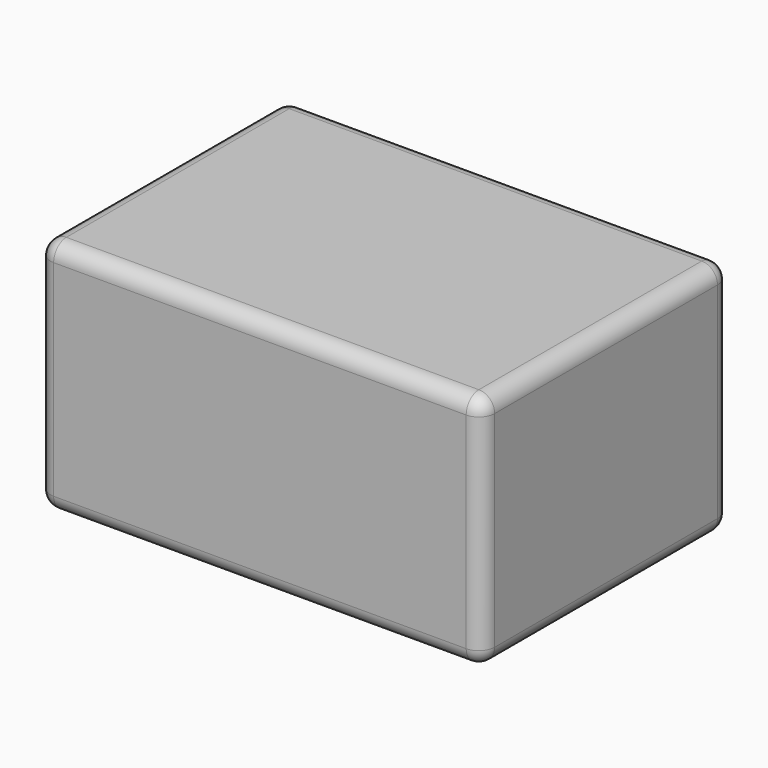
from build123d import *

# Parameters (mm, degrees)
F0_W         = 140.3584312648
F0_H         = 98.0234518647
F1_DEPTH     = 25
F2_DEPTH     = 50
F3_DEPTH     = 25
F4_R         = 5
F5_T1_DEPTH  = 65
F5_S5_W      = 5
F5_S5_H      = 5
F5_T6_DEPTH  = 5
F5_S11_W     = 5
F5_S11_H     = 5
F5_T12_DEPTH = 5
F5_S17_W     = 5
F5_S17_H     = 5
F5_T18_DEPTH = 5
F5_S23_W     = 5
F5_S23_H     = 5
F5_T24_DEPTH = 5
F5_S29_W     = 5
F5_S29_H     = 5
F5_T30_DEPTH = 5
F5_S35_W     = 5
F5_S35_H     = 5
F5_T36_DEPTH = 5
F5_S41_W     = 5
F5_S41_H     = 5
F5_T42_DEPTH = 5
F5_S47_W     = 5
F5_S47_H     = 5
F5_T48_DEPTH = 5


# Not quite as in the source:
# - a fillet or chamfer that OpenCascade refuses, or shapes differently, is made with other operations: its cross-section is extruded or revolved along the edge and cut away or added


with BuildPart() as f1:
    # F0 (on Top) → F1 (new body)
    with BuildSketch(Plane.XY):
        with Locations((-51.4516541734, -13.0883678794)):
            Rectangle(F0_W, F0_H)
    extrude(amount=F1_DEPTH)

    # F2 (add): a face of the model
    f2_faces = [f1.faces().sort_by_distance(p)[0] for p in [
        (-51.4516541734, -13.0883678794, 0),
    ]]
    extrude(f2_faces, amount=F2_DEPTH)

    # F3 (add): a face of the model
    f3_faces = [f1.faces().sort_by_distance(p)[0] for p in [
        (-51.4516541734, -13.0883678794, -50),
    ]]
    extrude(f3_faces, amount=-F3_DEPTH)

    # F4
    f4_edges = [f1.edges().sort_by_distance(p)[0] for p in [
        (18.727561, -13.088368, 25),
        (-121.63087, -13.088368, 25),
        (-51.451654, 35.923358, 25),
        (-51.451654, -62.100094, 25),
        (-51.451654, 35.923358, -50),
        (-121.63087, -13.088368, -50),
        (-51.451654, -62.100094, -50),
        (18.727561, -13.088368, -50),
    ]]
    fillet(f4_edges, radius=F4_R)

    # F5: fillet of radius 5 on 4 edges, made by hand

    # F5_s2 → F5_t1 (cut)
    with BuildSketch(Plane.XY.offset(-45)):
        with BuildLine():
            ThreePointArc((-116.6308698058, 35.923358053), (-120.1664037117, 34.4588919589), (-121.6308698058, 30.923358053))
            Line((-121.6308698058, 30.923358053), (-121.6308698058, 35.923358053))
            Line((-121.6308698058, 35.923358053), (-116.6308698058, 35.923358053))
        make_face()
        with BuildLine():
            ThreePointArc((13.7275614589, 35.923358053), (17.2630953649, 34.4588919589), (18.7275614589, 30.923358053))
            Line((18.7275614589, 30.923358053), (18.7275614589, 35.923358053))
            Line((18.7275614589, 35.923358053), (13.7275614589, 35.923358053))
        make_face()
        with BuildLine():
            ThreePointArc((18.7275614589, -57.1000938118), (17.2630953649, -60.6356277177), (13.7275614589, -62.1000938118))
            Line((13.7275614589, -62.1000938118), (18.7275614589, -62.1000938118))
            Line((18.7275614589, -62.1000938118), (18.7275614589, -57.1000938118))
        make_face()
        with BuildLine():
            ThreePointArc((-121.6308698058, -57.1000938118), (-120.1664037117, -60.6356277177), (-116.6308698058, -62.1000938118))
            Line((-116.6308698058, -62.1000938118), (-121.6308698058, -62.1000938118))
            Line((-121.6308698058, -62.1000938118), (-121.6308698058, -57.1000938118))
        make_face()
    extrude(amount=F5_T1_DEPTH, mode=Mode.SUBTRACT)


with BuildPart() as f5_tool4:
    # F5_s5 → F5_t6 (new body)
    with BuildSketch(Plane.YZ.offset(-116.6308698058)):
        with Locations((-59.6000938118, -47.5)):
            Rectangle(F5_S5_W, F5_S5_H)
    extrude(amount=-F5_T6_DEPTH)

    # F5_s7 → F5_t8 (revolve, cut)
    with BuildSketch(Plane(origin=(-116.6308698058, -57.1000938118, -45), x_dir=(0, 0.7071067812, 0.7071067812), z_dir=(0, -0.7071067812, 0.7071067812))):
        with BuildLine():
            ThreePointArc((0, -5), (5, 0), (0, 5))
            Line((0, 5), (0, -5))
        make_face()
    revolve(axis=Axis((-116.6308698058, -57.1000938118, -45), (-1, 0, 0)), mode=Mode.SUBTRACT)


with BuildPart() as f1_1:
    add(f1.part)

    # F5_t3: cut F5_tool4
    add(f5_tool4.part, mode=Mode.SUBTRACT)


with BuildPart() as f5_tool10:
    # F5_s11 → F5_t12 (new body)
    with BuildSketch(Plane.YZ.offset(-116.6308698058)):
        with Locations((-59.6000938118, 22.5)):
            Rectangle(F5_S11_W, F5_S11_H)
    extrude(amount=-F5_T12_DEPTH)

    # F5_s13 → F5_t14 (revolve, cut)
    with BuildSketch(Plane(origin=(-116.6308698058, -57.1000938118, 20), x_dir=(0, 0.7071067812, -0.7071067812), z_dir=(0, 0.7071067812, 0.7071067812))):
        with BuildLine():
            ThreePointArc((0, -5), (5, 0), (0, 5))
            Line((0, 5), (0, -5))
        make_face()
    revolve(axis=Axis((-116.6308698058, -57.1000938118, 20), (-1, 0, 0)), mode=Mode.SUBTRACT)


with BuildPart() as f1_2:
    add(f1_1.part)

    # F5_t9: cut F5_tool10
    add(f5_tool10.part, mode=Mode.SUBTRACT)


with BuildPart() as f5_tool16:
    # F5_s17 → F5_t18 (new body)
    with BuildSketch(Plane.YZ.offset(13.7275614589)):
        with Locations((-59.6000938118, 22.5)):
            Rectangle(F5_S17_W, F5_S17_H)
    extrude(amount=F5_T18_DEPTH)

    # F5_s19 → F5_t20 (revolve, cut)
    with BuildSketch(Plane(origin=(13.7275614589, -57.1000938118, 20), x_dir=(0, 0.7071067812, -0.7071067812), z_dir=(0, -0.7071067812, -0.7071067812))):
        with BuildLine():
            ThreePointArc((0, -5), (5, 0), (0, 5))
            Line((0, 5), (0, -5))
        make_face()
    revolve(axis=Axis((13.7275614589, -57.1000938118, 20), (1, 0, 0)), mode=Mode.SUBTRACT)


with BuildPart() as f1_3:
    add(f1_2.part)

    # F5_t15: cut F5_tool16
    add(f5_tool16.part, mode=Mode.SUBTRACT)


with BuildPart() as f5_tool22:
    # F5_s23 → F5_t24 (new body)
    with BuildSketch(Plane.YZ.offset(13.7275614589)):
        with Locations((-59.6000938118, -47.5)):
            Rectangle(F5_S23_W, F5_S23_H)
    extrude(amount=F5_T24_DEPTH)

    # F5_s25 → F5_t26 (revolve, cut)
    with BuildSketch(Plane(origin=(13.7275614589, -57.1000938118, -45), x_dir=(0, 0.7071067812, 0.7071067812), z_dir=(0, 0.7071067812, -0.7071067812))):
        with BuildLine():
            ThreePointArc((0, -5), (5, 0), (0, 5))
            Line((0, 5), (0, -5))
        make_face()
    revolve(axis=Axis((13.7275614589, -57.1000938118, -45), (1, 0, 0)), mode=Mode.SUBTRACT)


with BuildPart() as f1_4:
    add(f1_3.part)

    # F5_t21: cut F5_tool22
    add(f5_tool22.part, mode=Mode.SUBTRACT)


with BuildPart() as f5_tool28:
    # F5_s29 → F5_t30 (new body)
    with BuildSketch(Plane.XZ.offset(-30.923358053)):
        with Locations((16.2275614589, 22.5)):
            Rectangle(F5_S29_W, F5_S29_H)
    extrude(amount=-F5_T30_DEPTH)

    # F5_s31 → F5_t32 (revolve, cut)
    with BuildSketch(Plane(origin=(13.7275614589, 30.923358053, 20), x_dir=(-0.7071067812, 0, -0.7071067812), z_dir=(0.7071067812, 0, -0.7071067812))):
        with BuildLine():
            ThreePointArc((0, -5), (5, 0), (0, 5))
            Line((0, 5), (0, -5))
        make_face()
    revolve(axis=Axis((13.7275614589, 30.923358053, 20), (0, 1, 0)), mode=Mode.SUBTRACT)


with BuildPart() as f1_5:
    add(f1_4.part)

    # F5_t27: cut F5_tool28
    add(f5_tool28.part, mode=Mode.SUBTRACT)


with BuildPart() as f5_tool34:
    # F5_s35 → F5_t36 (new body)
    with BuildSketch(Plane.XZ.offset(-30.923358053)):
        with Locations((16.2275614589, -47.5)):
            Rectangle(F5_S35_W, F5_S35_H)
    extrude(amount=-F5_T36_DEPTH)

    # F5_s37 → F5_t38 (revolve, cut)
    with BuildSketch(Plane(origin=(13.7275614589, 30.923358053, -45), x_dir=(-0.7071067812, 0, 0.7071067812), z_dir=(-0.7071067812, 0, -0.7071067812))):
        with BuildLine():
            ThreePointArc((0, -5), (5, 0), (0, 5))
            Line((0, 5), (0, -5))
        make_face()
    revolve(axis=Axis((13.7275614589, 30.923358053, -45), (0, 1, 0)), mode=Mode.SUBTRACT)


with BuildPart() as f1_6:
    add(f1_5.part)

    # F5_t33: cut F5_tool34
    add(f5_tool34.part, mode=Mode.SUBTRACT)


with BuildPart() as f5_tool40:
    # F5_s41 → F5_t42 (new body)
    with BuildSketch(Plane.XZ.offset(-30.923358053)):
        with Locations((-119.1308698058, -47.5)):
            Rectangle(F5_S41_W, F5_S41_H)
    extrude(amount=-F5_T42_DEPTH)

    # F5_s43 → F5_t44 (revolve, cut)
    with BuildSketch(Plane(origin=(-116.6308698058, 30.923358053, -45), x_dir=(0.7071067812, 0, 0.7071067812), z_dir=(-0.7071067812, 0, 0.7071067812))):
        with BuildLine():
            ThreePointArc((0, -5), (5, 0), (0, 5))
            Line((0, 5), (0, -5))
        make_face()
    revolve(axis=Axis((-116.6308698058, 30.923358053, -45), (0, 1, 0)), mode=Mode.SUBTRACT)


with BuildPart() as f1_7:
    add(f1_6.part)

    # F5_t39: cut F5_tool40
    add(f5_tool40.part, mode=Mode.SUBTRACT)


with BuildPart() as f5_tool46:
    # F5_s47 → F5_t48 (new body)
    with BuildSketch(Plane.XZ.offset(-30.923358053)):
        with Locations((-119.1308698058, 22.5)):
            Rectangle(F5_S47_W, F5_S47_H)
    extrude(amount=-F5_T48_DEPTH)

    # F5_s49 → F5_t50 (revolve, cut)
    with BuildSketch(Plane(origin=(-116.6308698058, 30.923358053, 20), x_dir=(0.7071067812, 0, -0.7071067812), z_dir=(0.7071067812, 0, 0.7071067812))):
        with BuildLine():
            ThreePointArc((0, -5), (5, 0), (0, 5))
            Line((0, 5), (0, -5))
        make_face()
    revolve(axis=Axis((-116.6308698058, 30.923358053, 20), (0, 1, 0)), mode=Mode.SUBTRACT)


with BuildPart() as f1_8:
    add(f1_7.part)

    # F5_t45: cut F5_tool46
    add(f5_tool46.part, mode=Mode.SUBTRACT)


solid = f1_8.part
